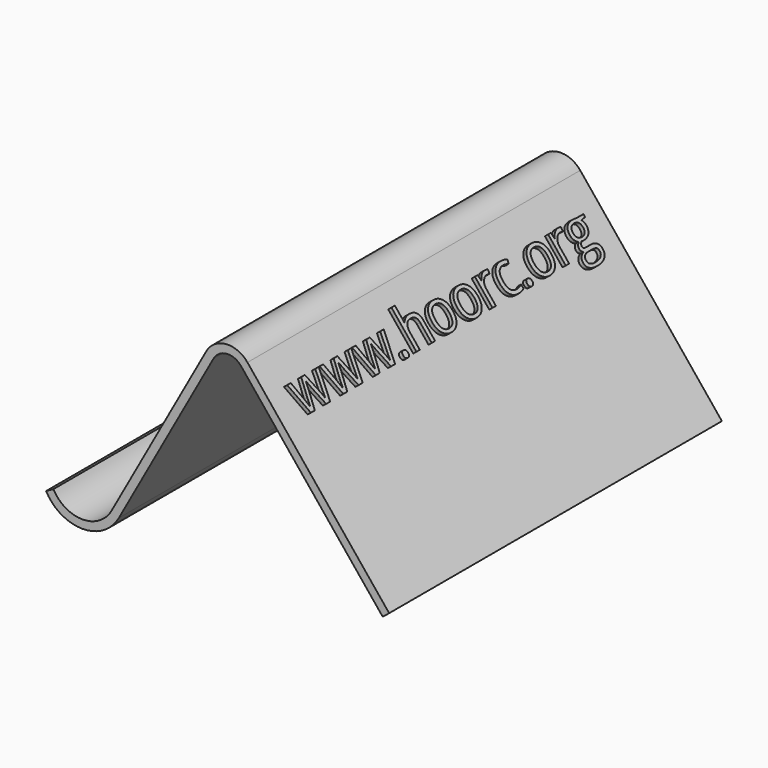
from build123d import *

# Parameters (mm, degrees)
F1_DEPTH     = 100
F2_TEXT_SIZE = 12.5471061058
F3_DEPTH     = 1


# Not quite as in the source:
# - Text() gives the source's letters only with a copy of the font that has no kerning and outlines rounded to 1/6400 em; it was checked with that copy


with BuildPart() as f1:
    # F0 (on Front) → F1 (new body)
    with BuildSketch(Plane.XZ):
        with BuildLine():
            Line((-4.3064132591, 41.1251087379), (-27.059993885, 0))
            ThreePointArc((-27.059993885, 0), (-34.0599741623, -4.1270501061), (-41.0599938849, -6.69048e-05))
            Line((-41.0599938849, -6.69048e-05), (-42.8099892577, -0.9683211044))
            ThreePointArc((-42.8099892577, -0.9683211044), (-34.0599646045, -6.1270501061), (-25.3099892579, -0.9682374734))
            Line((-25.3099892579, -0.9682374734), (-2.556408632, 40.1568712644))
            ThreePointArc((-2.556408632, 40.1568712644), (0.5918307745, 42.2048985417), (4.0501954715, 40.7401321058))
            Line((4.0501954715, 40.7401321058), (38.1160805471, -1.2598678942))
            Line((38.1160805471, -1.2598678942), (39.6693779717, 0))
            Line((39.6693779717, 0), (5.6034928961, 42))
            ThreePointArc((5.6034928961, 42), (0.4159458506, 44.1971496537), (-4.3064132591, 41.1251087379))
        make_face()
    extrude(amount=F1_DEPTH)

    # F2 (on face) → F3 (join)
    with BuildSketch(Plane(origin=(23.9279032323, 0, 19.4077428955), x_dir=(0, 1, 0), z_dir=(0.7766487123, 0, 0.6299339471))):
        with Locations((-95, 14.9723613665)):
            Text('www.hoorc.org', F2_TEXT_SIZE, font='Open Sans', text_align=(TextAlign.LEFT, TextAlign.BOTTOM))
    extrude(amount=F3_DEPTH)


solid = f1.part
